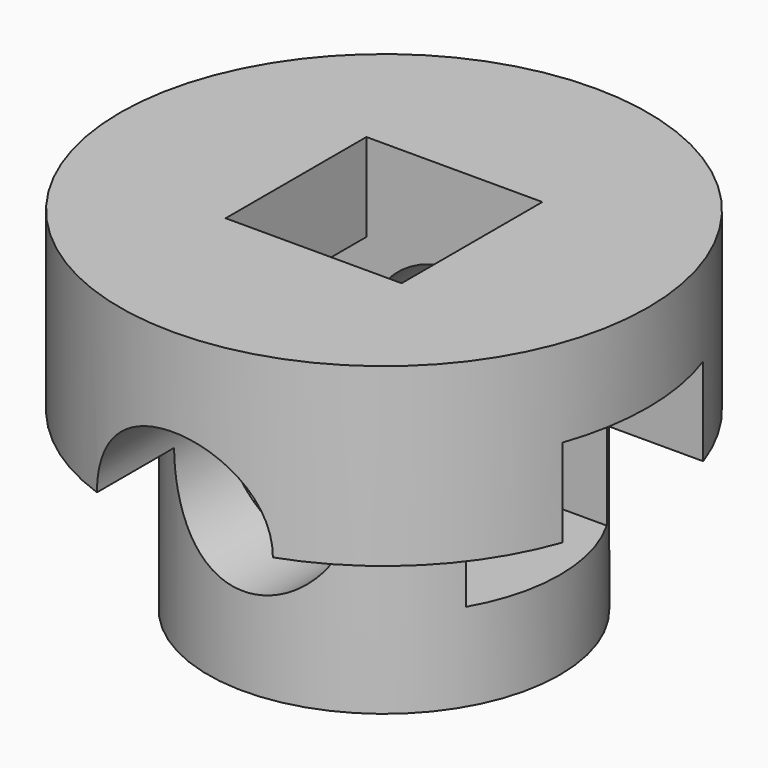
from build123d import *

# Parameters (mm, degrees)
F0_R      = 38.1
F1_DEPTH  = 25.4
F2_W      = 25.4
F2_H      = 25.4
F3_DEPTH  = 25.4
F4_R      = 25.4
F5_DEPTH  = 25.4
F6_W      = 25.4
F6_H      = 25.4
F7_DEPTH  = 166
F8_W      = 25.4
F8_H      = 25.4
F9_DEPTH  = 76.201
F10_R     = 12.7
F11_DEPTH = 38.101
F12_DEPTH = 50.8
F13_W     = 25.4
F13_H     = 25.4
F14_DEPTH = 38.1010001
F15_W     = 25.4
F15_H     = 25.4
F16_DEPTH = 50.8010001


# Not quite as in the source:
# - an extrude ends at something that could not be found from the text; its depth is read off the source's solid


with BuildPart() as f1:
    # F0 (on Top) → F1 (new body)
    with BuildSketch(Plane.XY):
        Circle(F0_R)
    extrude(amount=F1_DEPTH)

    # F2 (on face) → F3 (join)
    with BuildSketch(Plane.XY.offset(25.4)):
        Rectangle(F2_W, F2_H)
    extrude(amount=F3_DEPTH)

    # F4 (on face) → F5 (join)
    with BuildSketch(Plane(origin=(0, 0, 0), x_dir=(1, 0, 0), z_dir=(0, 0, -1))):
        Circle(F4_R)
    extrude(amount=F5_DEPTH)

    # F6 (on face) → F7 (cut, through all)
    with BuildSketch(Plane(origin=(0, 0, -25.4), x_dir=(1, 0, 0), z_dir=(0, 0, -1))):
        Rectangle(F6_W, F6_H)
    extrude(amount=F7_DEPTH, mode=Mode.SUBTRACT)

    # F8 (on face) → F9 (cut, through all)
    with BuildSketch(Plane(origin=(0, 0, -25.4), x_dir=(1, 0, 0), z_dir=(0, 0, -1))):
        Rectangle(F8_W, F8_H)
    extrude(amount=-F9_DEPTH, mode=Mode.SUBTRACT)

    # F10 (on Front) → F11 (cut, through all)
    with BuildSketch(Plane.XZ):
        Circle(F10_R)
    extrude(amount=-F11_DEPTH, mode=Mode.SUBTRACT)

    # F10 (on Front) → F12 (cut)
    with BuildSketch(Plane.XZ):
        Circle(F10_R)
    extrude(amount=F12_DEPTH, mode=Mode.SUBTRACT)

    # F13 (on Right) → F14 (cut, through all)
    with BuildSketch(Plane.YZ):
        Rectangle(F13_W, F13_H)
    extrude(amount=-F14_DEPTH, mode=Mode.SUBTRACT)

    # F15 (on face) → F16 (cut, through all)
    with BuildSketch(Plane.YZ.offset(-12.7)):
        Rectangle(F15_W, F15_H)
    extrude(amount=F16_DEPTH, mode=Mode.SUBTRACT)


solid = f1.part
